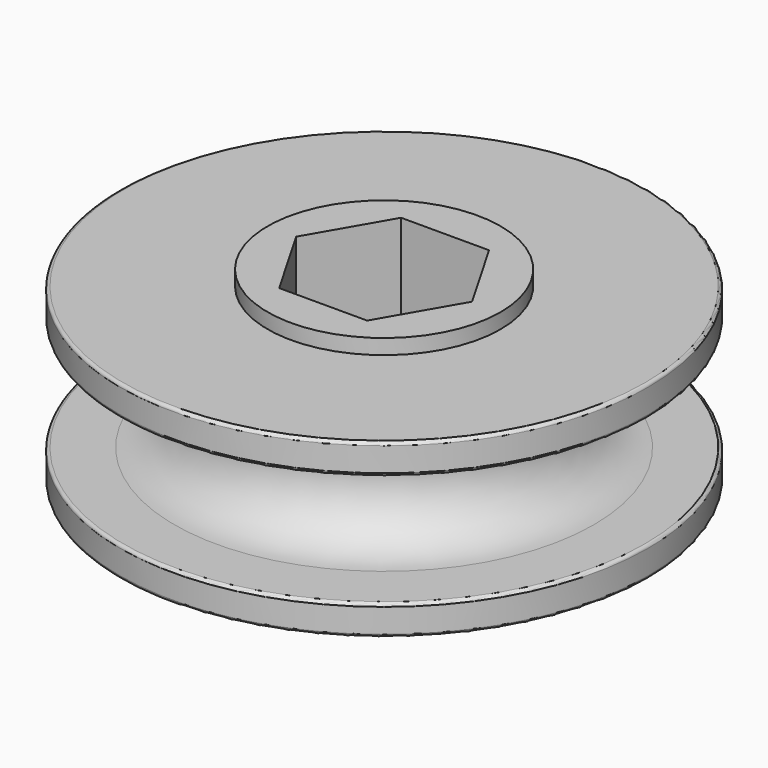
from build123d import *

# Parameters (mm, degrees)
F0_R     = 22.225
F1_DEPTH = 14.478
F4_R     = 9.8044812149
F5_DEPTH = 1.27
F7_R     = 0.254


# Not quite as in the source:
# - a pattern or mirror of a feature is missing from the dataset's text; its kind, count and spacing are read off the source's solid


with BuildPart() as f1:
    # F0 (on Top) → F1 (new body)
    with BuildSketch(Plane.XY):
        Circle(F0_R)
        Polygon((-7.4056719029, 0), (-3.7028359514, 6.4135), (3.7028359514, 6.4135), (7.4056719029, 0), (3.7028359514, -6.4135), (-3.7028359514, -6.4135), align=None, mode=Mode.SUBTRACT)
    extrude(amount=F1_DEPTH)

    # F2 (on Front) → F3 (revolve, cut)
    with BuildSketch(Plane.XZ):
        with BuildLine():
            Line((-22.225, 11.938), (-22.225, 2.54))
            Line((-22.225, 2.54), (-17.6526800774, 2.54))
            ThreePointArc((-17.6526800774, 2.54), (-12.9536800747, 7.2391599667), (-17.653, 11.938))
            Line((-17.653, 11.938), (-22.225, 11.938))
        make_face()
    revolve(axis=Axis((0, 0, 14.478), (0, 0, 1)), mode=Mode.SUBTRACT)

    # F4 (on face) → F5 (join)
    with BuildSketch(Plane.XY.offset(14.478)):
        Circle(F4_R)
        Polygon((-3.7028359514, 6.4135), (3.7028359514, 6.4135), (7.4056719029, 0), (3.7028359514, -6.4135), (-3.7028359514, -6.4135), (-7.4056719029, 0), align=None, mode=Mode.SUBTRACT)
    f5 = extrude(amount=F5_DEPTH)

    # F5_copies: F5 across plane
    add(f5.mirror(Plane(origin=(0, 0, 7.239), x_dir=(-1, 0, 0), z_dir=(0, 0, -1))))

    # F7
    f7_edges = [f1.edges().sort_by_distance(p)[0] for p in [
        (-22.225, 0, 0),
        (-22.225, 0, 14.478),
        (-22.225, 0, 11.938),
        (22.225, 0, 1.27),
        (-22.225, 0, 2.54),
    ]]
    fillet(f7_edges, radius=F7_R)


solid = f1.part
